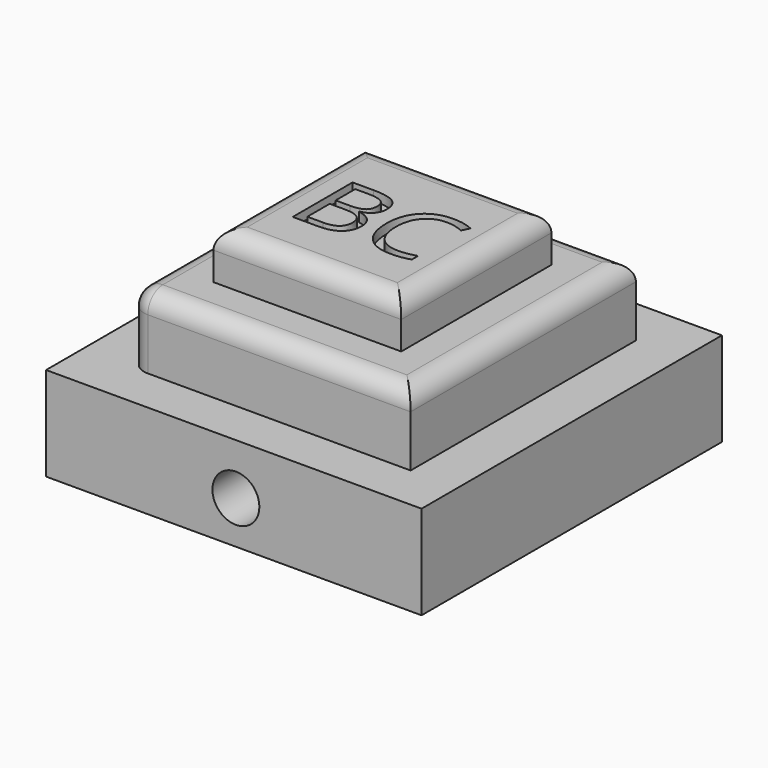
from build123d import *

# Parameters (mm, degrees)
F0_W          = 101.6
F0_H          = 101.6
F1_DEPTH      = 25.4
F2_W          = 76.2
F2_H          = 76.2
F3_DEPTH      = 19.05
F4_W          = 50.8
F4_H          = 50.8
F5_DEPTH      = 12.7
F6_R          = 6.35
F7_DEPTH      = 101.6
F8_R          = 5.08
F9_R          = 5.08
F10_R         = 5.08
F11_TEXT_SIZE = 28.3436228832
F12_DEPTH     = 2.54


# Not quite as in the source:
# - Text() gives the source's letters only with a copy of the font that has no kerning and outlines rounded to 1/6400 em; it was checked with that copy


with BuildPart() as f1:
    # F0 (on Top) → F1 (new body)
    with BuildSketch(Plane.XY):
        with Locations((50.8, 50.8)):
            Rectangle(F0_W, F0_H)
    extrude(amount=F1_DEPTH)

    # F6 (on face) → F7 (cut)
    with BuildSketch(Plane.XZ):
        with Locations((51.3604171574, 11.5625364706)):
            Circle(F6_R)
    extrude(amount=-F7_DEPTH, mode=Mode.SUBTRACT)


with BuildPart() as f3:
    # F2 (on face) → F3 (new body)
    with BuildSketch(Plane.XY.offset(25.4)):
        with Locations((50.7749388926, 50.3101658675)):
            Rectangle(F2_W, F2_H)
    extrude(amount=F3_DEPTH)

    # F8
    f8_edges = [f3.edges().sort_by_distance(p)[0] for p in [
        (12.674939, 50.310166, 44.45),
    ]]
    fillet(f8_edges, radius=F8_R)

    # F9
    f9_edges = [f3.edges().sort_by_distance(p)[0] for p in [
        (88.874939, 50.310166, 44.45),
        (53.314939, 88.410166, 44.45),
        (17.754939, 50.310166, 44.45),
        (53.314939, 12.210166, 44.45),
    ]]
    fillet(f9_edges, radius=F9_R)


with BuildPart() as f5:
    # F4 (on face) → F5 (new body)
    with BuildSketch(Plane.XY.offset(44.45)):
        with Locations((50.7749388926, 50.3101658675)):
            Rectangle(F4_W, F4_H)
    extrude(amount=F5_DEPTH)

    # F10
    f10_edges = [f5.edges().sort_by_distance(p)[0] for p in [
        (50.774939, 24.910166, 57.15),
        (76.174939, 50.310166, 57.15),
        (50.774939, 75.710166, 57.15),
        (25.374939, 50.310166, 57.15),
    ]]
    fillet(f10_edges, radius=F10_R)

    # F11 (on face) → F12 (cut)
    with BuildSketch(Plane.XY.offset(57.15)):
        with Locations((32.2571024299, 39.6264456213)):
            Text('BC', F11_TEXT_SIZE, font='Open Sans', text_align=(TextAlign.LEFT, TextAlign.BOTTOM))
    extrude(amount=-F12_DEPTH, mode=Mode.SUBTRACT)


solid = Compound([f1.part, f3.part, f5.part])
